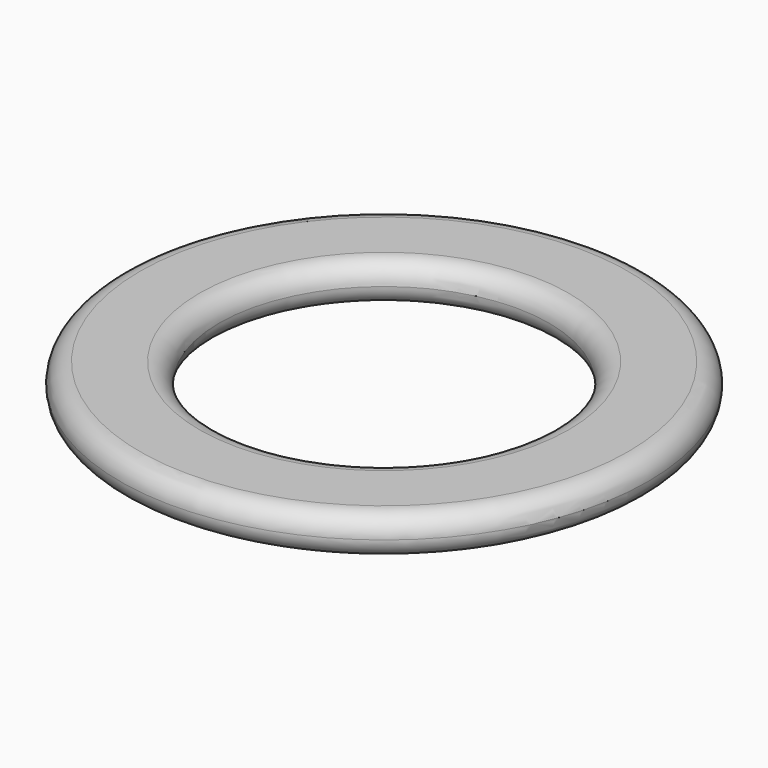
from build123d import *

# Parameters (mm, degrees)
F0_R     = 20
F0_R_2   = 12.5
F1_DEPTH = 3
F2_R     = 1.49999


# Not quite as in the source:
# - a fillet or chamfer is up to 0.001 mm smaller than in the source, because OpenCascade refuses the exact size


with BuildPart() as f1:
    # F0 (on Top) → F1 (new body)
    with BuildSketch(Plane.XY):
        Circle(F0_R)
        Circle(F0_R_2, mode=Mode.SUBTRACT)
    extrude(amount=F1_DEPTH)

    # F2 (radius 1.5 in the source; OpenCascade refuses exactly that, so slightly less here)
    f2_edges = [f1.edges().sort_by_distance(p)[0] for p in [
        (-20, 0, 3),
        (-12.5, 0, 3),
        (-12.5, 0, 0),
        (-20, 0, 0),
    ]]
    fillet(f2_edges, radius=F2_R)


solid = f1.part
